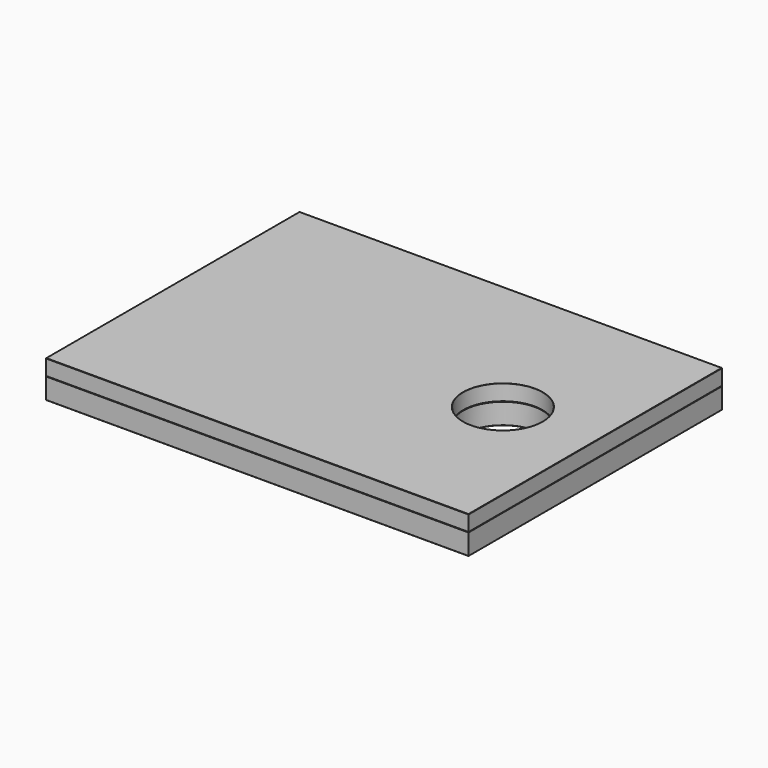
from build123d import *

# Parameters (mm, degrees)
F0_R      = 75
F1_DEPTH  = 40
F3_W      = 800
F3_H      = 600
F3_W_2    = 720
F3_H_2    = 520
F3_R      = 75
F4_DEPTH  = 30
F5_SIZE   = 0.5
F6_D      = 10
F6_DEPTH  = 20
F6_TIP    = 3.0043030951
F7_SIZE   = 0.5
F7_2_SIZE = 0.5


# Not quite as in the source:
# - a feature names something its author has since deleted; it is built from what else it names


with BuildPart() as f1:
    # F0 (on Top) → F1 (new body)
    with BuildSketch(Plane.XY):
        with BuildLine():
            Line((330, 75), (350, 75))
            Line((350, 75), (350, 300))
            Line((350, 300), (-450, 300))
            Line((-450, 300), (-450, 75))
            Line((-450, 75), (-430, 75))
            ThreePointArc((-430, 75), (-422.9289321881, 72.0710678119), (-420, 65))
            Line((-420, 65), (-420, 0))
            Line((-420, 0), (-420, -65))
            ThreePointArc((-420, -65), (-422.9289321881, -72.0710678119), (-430, -75))
            Line((-430, -75), (-450, -75))
            Line((-450, -75), (-450, -300))
            Line((-450, -300), (350, -300))
            Line((350, -300), (350, -75))
            Line((350, -75), (330, -75))
            ThreePointArc((330, -75), (322.9289321881, -72.0710678119), (320, -65))
            Line((320, -65), (320, 65))
            ThreePointArc((320, 65), (322.9289321881, 72.0710678119), (330, 75))
        make_face()
        with Locations((175, 0)):
            Circle(F0_R, mode=Mode.SUBTRACT)
        with BuildLine():
            Line((350, -75), (350, 75))
            Line((350, 75), (330, 75))
            ThreePointArc((330, 75), (322.9289321881, 72.0710678119), (320, 65))
            Line((320, 65), (320, -65))
            ThreePointArc((320, -65), (322.9289321881, -72.0710678119), (330, -75))
            Line((330, -75), (350, -75))
        make_face()
        with BuildLine():
            Line((-450, 0), (-450, -75))
            Line((-450, -75), (-430, -75))
            ThreePointArc((-430, -75), (-422.9289321881, -72.0710678119), (-420, -65))
            Line((-420, -65), (-420, 0))
            Line((-420, 0), (-450, 0))
        make_face()
        with BuildLine():
            Line((-430, 75), (-450, 75))
            Line((-450, 75), (-450, 0))
            Line((-450, 0), (-420, 0))
            Line((-420, 0), (-420, 65))
            ThreePointArc((-420, 65), (-422.9289321881, 72.0710678119), (-430, 75))
        make_face()
    extrude(amount=F1_DEPTH)

    # F7
    f7_edges = [f1.edges().sort_by_distance(p)[0] for p in [
        (-50, -300, 40),
        (350, 0, 40),
        (-50, 300, 40),
        (-450, 0, 40),
        (100, 0, 40),
        (-450, -300, 20),
        (350, -300, 20),
        (-50, -300, 0),
        (350, 300, 20),
        (-450, 300, 20),
        (-50, 300, 0),
        (350, 0, 0),
        (-450, 0, 0),
        (100, 0, 0),
    ]]
    chamfer(f7_edges, length=F7_SIZE)


with BuildPart() as f4:
    # F3 (on face) → F4 (new body)
    with BuildSketch(Plane.XY.offset(40)):
        with Locations((-50, 0)):
            Rectangle(F3_W, F3_H)
        with Locations((-50, 0)):
            Rectangle(F3_W_2, F3_H_2, mode=Mode.SUBTRACT)
        with Locations((-50, 0)):
            Rectangle(F3_W_2, F3_H_2)
        with Locations((175, 0)):
            Circle(F3_R, mode=Mode.SUBTRACT)
    extrude(amount=F4_DEPTH)

    # F5
    f5_edges = [f4.edges().sort_by_distance(p)[0] for p in [
        (-50, 300, 70),
        (-450, 0, 70),
        (-50, -300, 70),
        (350, 0, 70),
        (100, 0, 70),
        (-50, 300, 40),
        (-450, 0, 40),
        (-50, -300, 40),
        (350, 0, 40),
        (100, 0, 40),
        (350, 300, 55),
        (-450, 300, 55),
        (-450, -300, 55),
        (350, -300, 55),
    ]]
    chamfer(f5_edges, length=F5_SIZE)

    # F6
    with Locations(Plane(origin=(0, 0, 40), x_dir=(1, 0, 0), z_dir=(0, 0, -1))):
        with Locations((-410, -260), (310, -260), (310, 260), (-410, 260)):
            Hole(F6_D / 2, depth=F6_DEPTH)
            with Locations((0, 0, -(F6_DEPTH + F6_TIP / 2))):  # 118° drill point
                Cone(0, F6_D / 2, F6_TIP, mode=Mode.SUBTRACT)

    # F7#2
    f7_2_edges = [f4.edges().sort_by_distance(p)[0] for p in [
        (100, 0, 69.5),
    ]]
    chamfer(f7_2_edges, length=F7_2_SIZE)


solid = Compound([f1.part, f4.part])
